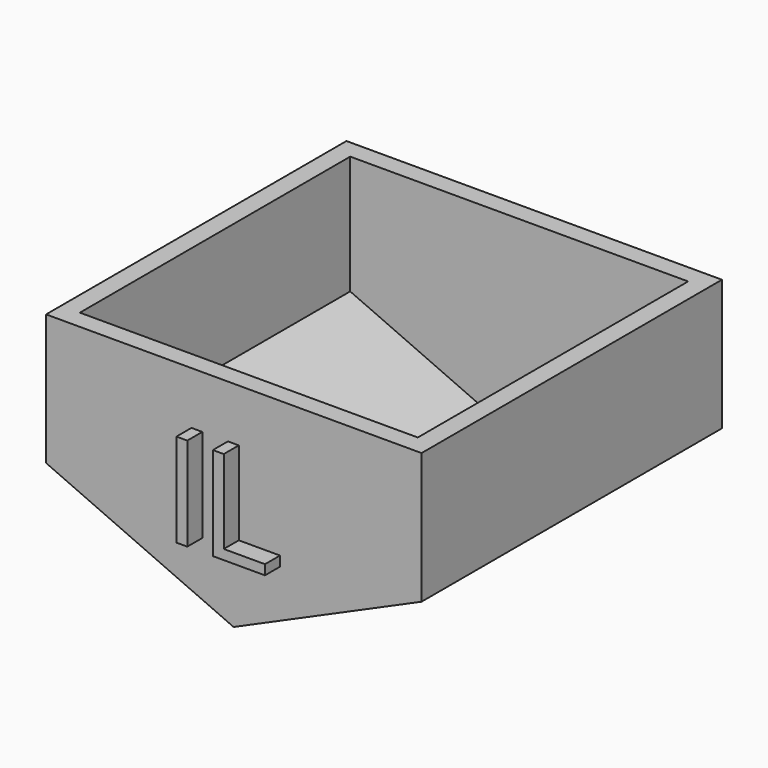
from build123d import *

# Parameters (mm, degrees)
F1_DEPTH     = 50.8
F2_T         = -2.54
F3_TEXT_SIZE = 17.7000083366
F4_DEPTH     = 2.54


# Not quite as in the source:
# - Text() gives the source's letters only with a copy of the font that has no kerning and outlines rounded to 1/6400 em; it was checked with that copy


with BuildPart() as f1:
    # F0 (on Front) → F1 (new body)
    with BuildSketch(Plane.XZ):
        Polygon((25.4366046359, 14.5336864816), (-25.3633953641, 14.5336864816), (-25.3633953641, -3.1716083297), (0, -14.4521969697), (25.4366046359, -3.1716083297), align=None)
    extrude(amount=F1_DEPTH)

    # F2
    f2_openings = [f1.faces().sort_by_distance(p)[0] for p in [
        (0.036605, -25.4, 14.533686),
    ]]
    offset(amount=F2_T, openings=f2_openings)

    # F3 (on face) → F4 (join)
    with BuildSketch(Plane.XZ.offset(50.8)):
        with Locations((-7.4312378751, -5.2263452671)):
            Text('IL', F3_TEXT_SIZE, font='Open Sans', text_align=(TextAlign.LEFT, TextAlign.BOTTOM))
    extrude(amount=F4_DEPTH)


solid = f1.part
